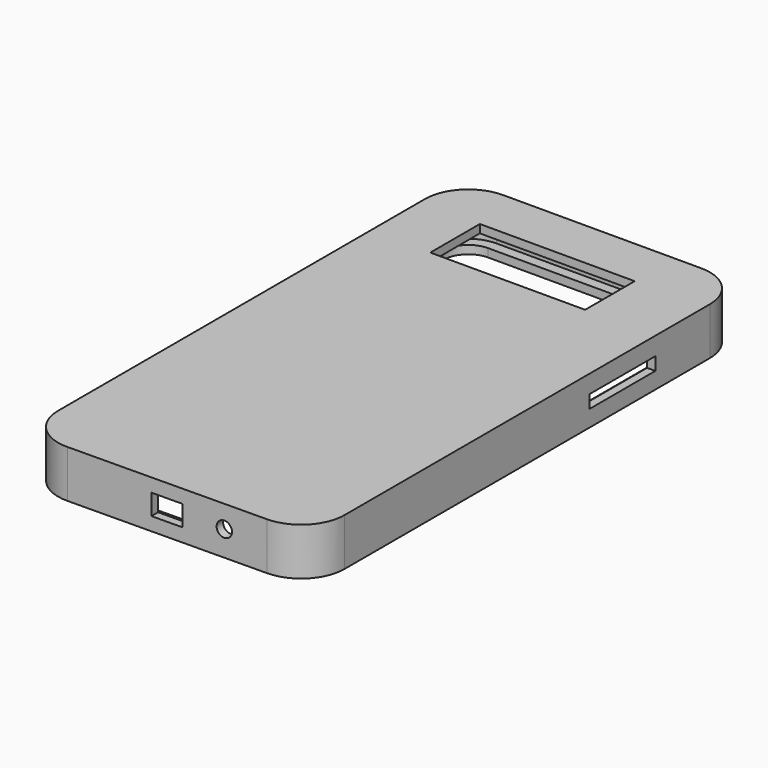
from build123d import *

# Parameters (mm, degrees)
F0_W       = 38.1
F0_H       = 15.24
F1_DEPTH   = 7.62
F2_W       = 20.32
F2_H       = 3.1982096843
F3_DEPTH   = 25.4
F5_W       = 10.16
F5_H       = 2.54
F6_DEPTH   = 25.4
F4_W       = 3.81
F4_H       = 5.08
F4_R       = 1.8758350377
F7_DEPTH   = 25.4
F8_DEPTH   = 7.62
F1_FACE3_W = 38.1
F1_FACE3_H = 15.24
F9_DEPTH   = 2.032
F10_DEPTH  = 2.032


with BuildPart() as f1:
    # F0 (on Top) → F1 (new body)
    with BuildSketch(Plane.XY):
        with BuildLine():
            Line((15.0151342493, 51.7147295177), (-33.7528657507, 51.7147295177))
            ThreePointArc((-33.7528657507, 51.7147295177), (-39.8594399131, 49.18530368), (-42.3888657507, 43.0787295177))
            Line((-42.3888657507, 43.0787295177), (-42.3888657507, -69.7396477934))
            ThreePointArc((-42.3888657507, -69.7396477934), (-39.8300752503, -75.8754460869), (-33.6700096372, -78.3752503123))
            Line((-33.6700096372, -78.3752503123), (15.0979903628, -77.9073354291))
            ThreePointArc((15.0979903628, -77.9073354291), (21.1509325427, -75.3489424097), (23.6511342493, -69.2717329101))
            Line((23.6511342493, -69.2717329101), (23.6511342493, 43.0787295177))
            ThreePointArc((23.6511342493, 43.0787295177), (21.1217084116, 49.18530368), (15.0151342493, 51.7147295177))
        make_face()
        with BuildLine():
            ThreePointArc((-39.8488657507, 43.0787295177), (-38.0633886888, 47.3892524558), (-33.7528657507, 49.1747295177))
            Line((-33.7528657507, 49.1747295177), (15.0151342493, 49.1747295177))
            ThreePointArc((15.0151342493, 49.1747295177), (19.3256571874, 47.3892524558), (21.1111342493, 43.0787295177))
            Line((21.1111342493, 43.0787295177), (21.1111342493, -69.2717329101))
            ThreePointArc((21.1111342493, -69.2717329101), (19.3462859858, -73.561527851), (15.0736209176, -75.3674523353))
            Line((15.0736209176, -75.3674523353), (-33.6943790824, -75.8353672185))
            ThreePointArc((-33.6943790824, -75.8353672185), (-38.0426606916, -74.07079953), (-39.8488657507, -69.7396477934))
            Line((-39.8488657507, -69.7396477934), (-39.8488657507, 43.0787295177))
        make_face(mode=Mode.SUBTRACT)
        with BuildLine():
            Line((15.0151342493, 49.1747295177), (-33.7528657507, 49.1747295177))
            ThreePointArc((-33.7528657507, 49.1747295177), (-38.0633886888, 47.3892524558), (-39.8488657507, 43.0787295177))
            Line((-39.8488657507, 43.0787295177), (-39.8488657507, -69.7396477934))
            ThreePointArc((-39.8488657507, -69.7396477934), (-38.0426606916, -74.07079953), (-33.6943790824, -75.8353672185))
            Line((-33.6943790824, -75.8353672185), (15.0736209176, -75.3674523353))
            ThreePointArc((15.0736209176, -75.3674523353), (19.3462859858, -73.561527851), (21.1111342493, -69.2717329101))
            Line((21.1111342493, -69.2717329101), (21.1111342493, 43.0787295177))
            ThreePointArc((21.1111342493, 43.0787295177), (19.3256571874, 47.3892524558), (15.0151342493, 49.1747295177))
        make_face()
        with Locations((-10.6388657507, 33.9347295177)):
            Rectangle(F0_W, F0_H, mode=Mode.SUBTRACT)
    extrude(amount=F1_DEPTH)

    # F2 (on face) → F3 (join)
    with BuildSketch(Plane.YZ.offset(23.6511342493)):
        with Locations((16.1547295177, 3.6192152184)):
            Rectangle(F2_W, F2_H)
    extrude(amount=F3_DEPTH)

    # F5 (on face) → F6 (join)
    with BuildSketch(Plane(origin=(-42.3888657507, 0, 0), x_dir=(0, -1, 0), z_dir=(-1, 0, 0))):
        with Locations((-8.5347295177, 4.0440695514)):
            Rectangle(F5_W, F5_H)
    extrude(amount=F6_DEPTH)

    # F4 (on face) → F7 (join)
    with BuildSketch(Plane(origin=(0.7488193587, -78.045011583, 0), x_dir=(0.9999539739, 0.0095942697, 0), z_dir=(0.0095942697, -0.9999539739, 0))):
        with Locations((-11.9402908808, 3.81)):
            Rectangle(F4_W, F4_H)
        with Locations((-8.1302908808, 3.81)):
            Rectangle(F4_W, F4_H)
        with Locations((3.9347091192, 4.1537573561)):
            Circle(F4_R)
    extrude(amount=F7_DEPTH)


with BuildPart() as f8:
    # F0 (on Top) → F8 (new body, through all)
    with BuildSketch(Plane.XY):
        with BuildLine():
            Line((15.0151342493, 53.7467295177), (-33.7528657507, 53.7467295177))
            ThreePointArc((-33.7528657507, 53.7467295177), (-41.2962808924, 50.6221446594), (-44.4208657507, 43.0787295177))
            Line((-44.4208657507, 43.0787295177), (-44.4208657507, -69.7396477934))
            ThreePointArc((-44.4208657507, -69.7396477934), (-41.2600068973, -77.3191633324), (-33.6505140811, -80.4071567873))
            Line((-33.6505140811, -80.4071567873), (15.1174859189, -79.9392419041))
            ThreePointArc((15.1174859189, -79.9392419041), (22.5946497883, -76.7788740567), (25.6831342493, -69.2717329101))
            Line((25.6831342493, -69.2717329101), (25.6831342493, 43.0787295177))
            ThreePointArc((25.6831342493, 43.0787295177), (22.558549391, 50.6221446594), (15.0151342493, 53.7467295177))
        make_face()
        with BuildLine():
            ThreePointArc((-42.3888657507, 43.0787295177), (-39.8594399131, 49.18530368), (-33.7528657507, 51.7147295177))
            Line((-33.7528657507, 51.7147295177), (15.0151342493, 51.7147295177))
            ThreePointArc((15.0151342493, 51.7147295177), (21.1217084116, 49.18530368), (23.6511342493, 43.0787295177))
            Line((23.6511342493, 43.0787295177), (23.6511342493, -69.2717329101))
            ThreePointArc((23.6511342493, -69.2717329101), (21.1509325427, -75.3489424097), (15.0979903628, -77.9073354291))
            Line((15.0979903628, -77.9073354291), (-33.6700096372, -78.3752503123))
            ThreePointArc((-33.6700096372, -78.3752503123), (-39.8300752503, -75.8754460869), (-42.3888657507, -69.7396477934))
            Line((-42.3888657507, -69.7396477934), (-42.3888657507, 43.0787295177))
        make_face(mode=Mode.SUBTRACT)
    extrude(amount=F8_DEPTH)

    # F8_face (on face) + F1_face3 (on face) → F9 (join)
    with BuildSketch(Plane(origin=(-9.4104092831, -13.214065849, 7.62), x_dir=(1, 0, 0), z_dir=(0, 0, 1))):
        with BuildLine():
            Line((35.0935435324, -56.0576670611), (35.0935435324, 56.2927953667))
            ThreePointArc((35.0935435324, 56.2927953667), (31.9689586741, 63.8362105084), (24.4255435324, 66.9607953667))
            Line((24.4255435324, 66.9607953667), (-24.3424564676, 66.9607953667))
            ThreePointArc((-24.3424564676, 66.9607953667), (-31.8858716093, 63.8362105084), (-35.0104564676, 56.2927953667))
            Line((-35.0104564676, 56.2927953667), (-35.0104564676, -56.5255819444))
            ThreePointArc((-35.0104564676, -56.5255819444), (-31.8495976142, -64.1050974834), (-24.240104798, -67.1930909383))
            Line((-24.240104798, -67.1930909383), (24.527895202, -66.7251760551))
            ThreePointArc((24.527895202, -66.7251760551), (32.0050590714, -63.5648082077), (35.0935435324, -56.0576670611))
        make_face()
        with BuildLine():
            ThreePointArc((-32.9784564676, 56.2927953667), (-30.4490306299, 62.399369529), (-24.3424564676, 64.9287953667))
            Line((-24.3424564676, 64.9287953667), (24.4255435324, 64.9287953667))
            ThreePointArc((24.4255435324, 64.9287953667), (30.5321176947, 62.399369529), (33.0615435324, 56.2927953667))
            Line((33.0615435324, 56.2927953667), (33.0615435324, -56.0576670611))
            ThreePointArc((33.0615435324, -56.0576670611), (30.5613418259, -62.1348765607), (24.5083996459, -64.69326958))
            Line((24.5083996459, -64.69326958), (-24.2596003541, -65.1611844633))
            ThreePointArc((-24.2596003541, -65.1611844633), (-30.4196659672, -62.6613802378), (-32.9784564676, -56.5255819444))
            Line((-32.9784564676, -56.5255819444), (-32.9784564676, 56.2927953667))
        make_face(mode=Mode.SUBTRACT)
    with BuildSketch(Plane(origin=(-9.3022040754, -16.6655356146, 7.62), x_dir=(1, 0, 0), z_dir=(0, 0, 1))):
        with BuildLine():
            ThreePointArc((32.9533383247, 59.7442651323), (30.423912487, 65.8508392946), (24.3173383247, 68.3802651323))
            Line((24.3173383247, 68.3802651323), (-24.4506616753, 68.3802651323))
            ThreePointArc((-24.4506616753, 68.3802651323), (-30.5572358376, 65.8508392946), (-33.0866616753, 59.7442651323))
            Line((-33.0866616753, 59.7442651323), (-33.0866616753, -53.0741121788))
            ThreePointArc((-33.0866616753, -53.0741121788), (-30.5278711749, -59.2099104723), (-24.3678055618, -61.7097146977))
            Line((-24.3678055618, -61.7097146977), (24.4001944382, -61.2417998145))
            ThreePointArc((24.4001944382, -61.2417998145), (30.4531366182, -58.6834067951), (32.9533383247, -52.6061972956))
            Line((32.9533383247, -52.6061972956), (32.9533383247, 59.7442651323))
        make_face()
        with Locations((-1.3366616753, 50.6002651323)):
            Rectangle(F1_FACE3_W, F1_FACE3_H, mode=Mode.SUBTRACT)
    extrude(amount=F9_DEPTH)

    # F0 (on Top) → F10 (join)
    with BuildSketch(Plane.XY):
        with BuildLine():
            Line((15.0151342493, 53.7467295177), (-33.7528657507, 53.7467295177))
            ThreePointArc((-33.7528657507, 53.7467295177), (-41.2962808924, 50.6221446594), (-44.4208657507, 43.0787295177))
            Line((-44.4208657507, 43.0787295177), (-44.4208657507, -69.7396477934))
            ThreePointArc((-44.4208657507, -69.7396477934), (-41.2600068973, -77.3191633324), (-33.6505140811, -80.4071567873))
            Line((-33.6505140811, -80.4071567873), (15.1174859189, -79.9392419041))
            ThreePointArc((15.1174859189, -79.9392419041), (22.5946497883, -76.7788740567), (25.6831342493, -69.2717329101))
            Line((25.6831342493, -69.2717329101), (25.6831342493, 43.0787295177))
            ThreePointArc((25.6831342493, 43.0787295177), (22.558549391, 50.6221446594), (15.0151342493, 53.7467295177))
        make_face()
        with BuildLine():
            ThreePointArc((-42.3888657507, 43.0787295177), (-39.8594399131, 49.18530368), (-33.7528657507, 51.7147295177))
            Line((-33.7528657507, 51.7147295177), (15.0151342493, 51.7147295177))
            ThreePointArc((15.0151342493, 51.7147295177), (21.1217084116, 49.18530368), (23.6511342493, 43.0787295177))
            Line((23.6511342493, 43.0787295177), (23.6511342493, -69.2717329101))
            ThreePointArc((23.6511342493, -69.2717329101), (21.1509325427, -75.3489424097), (15.0979903628, -77.9073354291))
            Line((15.0979903628, -77.9073354291), (-33.6700096372, -78.3752503123))
            ThreePointArc((-33.6700096372, -78.3752503123), (-39.8300752503, -75.8754460869), (-42.3888657507, -69.7396477934))
            Line((-42.3888657507, -69.7396477934), (-42.3888657507, 43.0787295177))
        make_face(mode=Mode.SUBTRACT)
        with BuildLine():
            Line((15.0151342493, 51.7147295177), (-33.7528657507, 51.7147295177))
            ThreePointArc((-33.7528657507, 51.7147295177), (-39.8594399131, 49.18530368), (-42.3888657507, 43.0787295177))
            Line((-42.3888657507, 43.0787295177), (-42.3888657507, -69.7396477934))
            ThreePointArc((-42.3888657507, -69.7396477934), (-39.8300752503, -75.8754460869), (-33.6700096372, -78.3752503123))
            Line((-33.6700096372, -78.3752503123), (15.0979903628, -77.9073354291))
            ThreePointArc((15.0979903628, -77.9073354291), (21.1509325427, -75.3489424097), (23.6511342493, -69.2717329101))
            Line((23.6511342493, -69.2717329101), (23.6511342493, 43.0787295177))
            ThreePointArc((23.6511342493, 43.0787295177), (21.1217084116, 49.18530368), (15.0151342493, 51.7147295177))
        make_face()
        with BuildLine():
            ThreePointArc((-39.8488657507, 43.0787295177), (-38.0633886888, 47.3892524558), (-33.7528657507, 49.1747295177))
            Line((-33.7528657507, 49.1747295177), (15.0151342493, 49.1747295177))
            ThreePointArc((15.0151342493, 49.1747295177), (19.3256571874, 47.3892524558), (21.1111342493, 43.0787295177))
            Line((21.1111342493, 43.0787295177), (21.1111342493, -69.2717329101))
            ThreePointArc((21.1111342493, -69.2717329101), (19.3462859858, -73.561527851), (15.0736209176, -75.3674523353))
            Line((15.0736209176, -75.3674523353), (-33.6943790824, -75.8353672185))
            ThreePointArc((-33.6943790824, -75.8353672185), (-38.0426606916, -74.07079953), (-39.8488657507, -69.7396477934))
            Line((-39.8488657507, -69.7396477934), (-39.8488657507, 43.0787295177))
        make_face(mode=Mode.SUBTRACT)
    extrude(amount=-F10_DEPTH)

    # F11: cut F1
    add(f1.part, mode=Mode.SUBTRACT)


solid = f8.part
